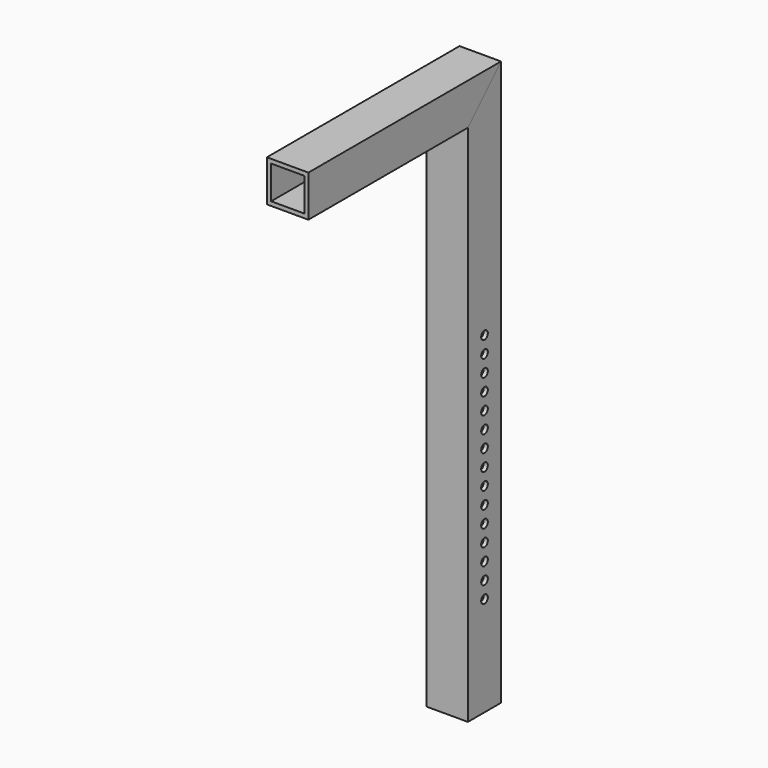
from build123d import *

# Parameters (mm, degrees)
F0_W      = 63.5
F0_H      = 63.5
F0_W_2    = 50.8
F0_H_2    = 50.8
F1_DEPTH  = 863.6
F3_DEPTH  = 63.5
F5_D      = 12.7
F6_W      = 63.5
F6_H      = 63.5
F6_W_2    = 50.8
F6_H_2    = 50.8
F7_DEPTH  = 368.3
F10_DEPTH = 63.5


# Not quite as in the source:
# - a length typed as a fraction of an inch, garbled in the dataset ("3 / 203.2 mm" for 3/8 in), is restored


with BuildPart() as f1:
    # F0 (on Top) → F1 (new body)
    with BuildSketch(Plane.XY):
        Rectangle(F0_W, F0_H)
        Rectangle(F0_W_2, F0_H_2, mode=Mode.SUBTRACT)
    extrude(amount=F1_DEPTH)

    # F2 (on face) → F3 (cut)
    with BuildSketch(Plane.YZ.offset(31.75)):
        Polygon((-31.75, 800.1), (31.75, 863.6), (-31.75, 863.6), align=None)
    extrude(amount=-F3_DEPTH, mode=Mode.SUBTRACT)

    # F5 (through all)
    with Locations(Plane.YZ.offset(31.75)):
        with Locations((0, 152.4), (0, 177.8), (0, 203.2), (0, 228.6), (0, 254), (0, 279.4), (0, 304.8), (0, 330.2), (0, 355.6), (0, 381), (0, 431.8), (0, 406.4), (0, 457.2), (0, 482.6), (0, 508)):
            Hole(F5_D / 2)


with BuildPart() as f7:
    # F6 (on Front) → F7 (new body)
    with BuildSketch(Plane.XZ):
        with Locations((-0.1429180503, -31.75)):
            Rectangle(F6_W, F6_H)
        with Locations((0, -31.75)):
            Rectangle(F6_W_2, F6_H_2, mode=Mode.SUBTRACT)
    extrude(amount=F7_DEPTH)


with BuildPart() as f7_1:
    # F8: moved
    add(f7.part.moved(Location((0, 31.75, 0))))

    # F9 (on face) → F10 (cut)
    with BuildSketch(Plane(origin=(-31.8929180503, 0, 0), x_dir=(0, -1, 0), z_dir=(-1, 0, 0))):
        Polygon((31.75, -63.5), (-31.75, 0), (-31.75, -63.5), align=None)
    extrude(amount=-F10_DEPTH, mode=Mode.SUBTRACT)


with BuildPart() as f7_2:
    # F11: moved
    add(f7_1.part.moved(Location((0, 0, 863.6))))


solid = Compound([f1.part, f7_2.part])
